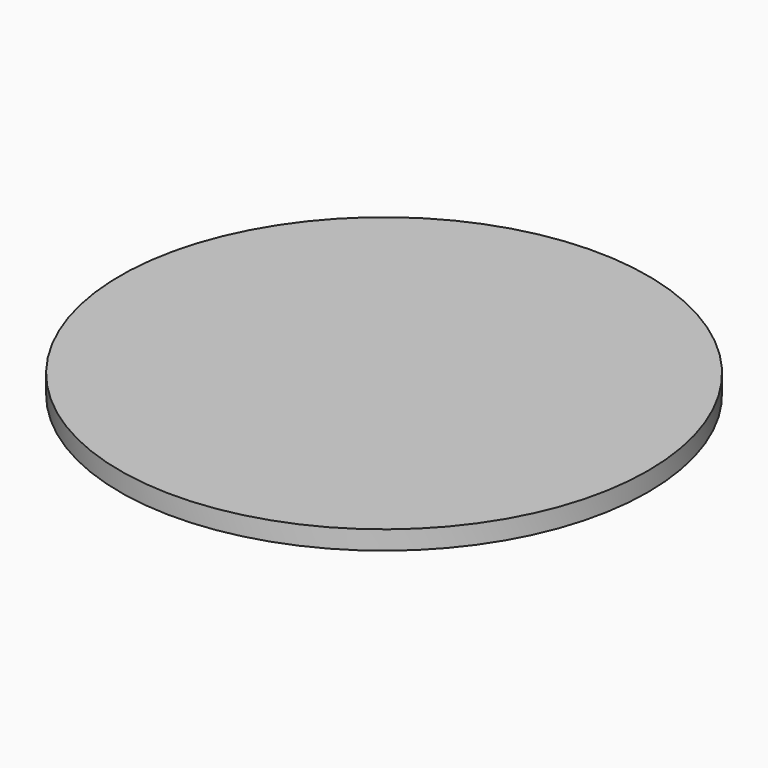
from build123d import *

# Parameters (mm, degrees)
F0_R            = 2.25
F1_DEPTH        = 2
F1_TAPER        = 3
F2_R            = 7
F3_DEPTH        = 0.5
F5_R            = 0.15
F6_DEPTH        = 0.1
F6_COPIES_COUNT = 4


# Not quite as in the source:
# - a pattern or mirror of a feature is missing from the dataset's text; its kind, count and spacing are read off the source's solid


with BuildPart() as f1:
    # F0 (on Top) → F1 (new body)
    with BuildSketch(Plane.XY):
        Circle(F0_R)
    extrude(amount=-F1_DEPTH, taper=F1_TAPER)

    # F2 (on Top) → F3 (join)
    with BuildSketch(Plane.XY):
        Circle(F2_R)
    extrude(amount=F3_DEPTH)


with BuildPart() as f1_1:
    # F4: moved
    add(f1.part.moved(Location((0, 0, 0.1))))

    # F5 (on Top) → F6 (join)
    with BuildSketch(Plane.XY):
        with Locations((-4, 0)):
            Circle(F5_R)
    f6 = extrude(amount=F6_DEPTH)

    # F6_copies: F6 ×4 about axis
    f6_copies_axis = Axis((0, 0, 0), (0, 0, 1))
    for i in range(1, F6_COPIES_COUNT):
        add(f6.rotate(f6_copies_axis, i * 360 / F6_COPIES_COUNT))


solid = f1_1.part
